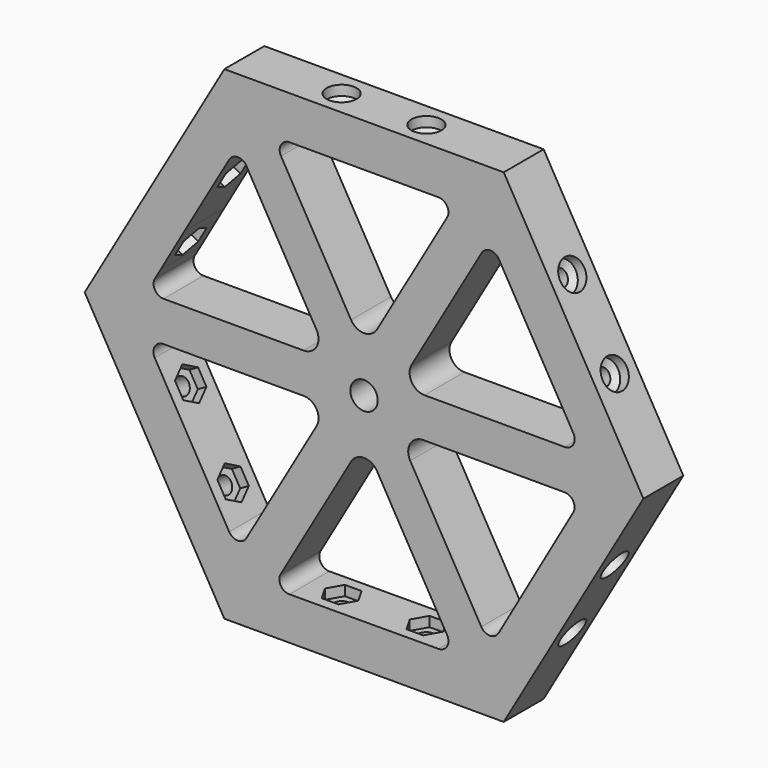
from build123d import *

# Parameters (mm, degrees)
F0_R      = 4
F1_DEPTH  = 3
F2_DEPTH  = 10
F8_D      = 6
F8_DEPTH  = 2
F8_TIP    = 1.8025818571
F9_D      = 3.3
F9_DEPTH  = 13.5
F9_START  = 2.8111618
F9_TIP    = 0.9914200214
F10_D     = 3.3
F10_DEPTH = 13.5
F10_TIP   = 0.9914200214
F11_D     = 6
F11_DEPTH = 2
F11_TIP   = 1.8025818571
F12_D     = 6
F12_DEPTH = 2
F12_TIP   = 1.8025818571
F13_D     = 3.3
F13_DEPTH = 13.5
F13_START = 2.8111618
F13_TIP   = 0.9914200214
F15_D     = 3.3
F15_DEPTH = 13.5
F15_TIP   = 0.9914200214
F16_D     = 6
F16_DEPTH = 2
F16_TIP   = 1.8025818571
F17_D     = 6
F17_DEPTH = 2
F17_TIP   = 1.8025818571
F18_D     = 3.3
F18_DEPTH = 13.5
F18_START = 2.8111618
F18_TIP   = 0.9914200214
F19_D     = 3.3
F19_DEPTH = 13.5
F19_TIP   = 0.9914200214
F20_D     = 6
F20_DEPTH = 2
F20_TIP   = 1.8025818571
F22_DEPTH = 2
F24_DEPTH = 2
F25_R     = 1.65
F26_DEPTH = 2
F28_DEPTH = 2
F29_R     = 1.65
F30_DEPTH = 2
F32_DEPTH = 2
F34_DEPTH = 2
F35_D     = 5.5
F35_DEPTH = 15.81
F35_TIP   = 1.6523667023


# Not quite as in the source:
# - a feature names something its author has since deleted; it is built from what else it names


with BuildPart() as f1:
    # F0 (on Front) → F1 (new body)
    with BuildSketch(Plane.XZ):
        Polygon((28, -48.4974226119), (56, 0), (28, 48.4974226119), (-28, 48.4974226119), (-56, 0), (-28, -48.4974226119), align=None)
        with BuildLine():
            ThreePointArc((-2.5980762114, -12.5), (0, -11), (2.5980762114, -12.5))
            Line((2.5980762114, -12.5), (16.6589147242, -36.8540867013))
            ThreePointArc((16.6589147242, -36.8540867013), (16.6605005999, -38.8513348401), (14.9332161477, -39.8540766136))
            Line((14.9332161477, -39.8540766136), (-14.9735632922, -39.9490644792))
            ThreePointArc((-14.9735632922, -39.9490644792), (-16.7117197395, -38.9526061697), (-16.7137597469, -36.9490810672))
            Line((-16.7137597469, -36.9490810672), (-2.5980762114, -12.5))
        make_face(mode=Mode.SUBTRACT)
        with BuildLine():
            ThreePointArc((-23.5773502692, -32.8371685741), (-25.3094010768, -33.8371685741), (-27.0414518843, -32.8371685741))
            Line((-27.0414518843, -32.8371685741), (-41.9585481157, -7))
            ThreePointArc((-41.9585481157, -7), (-41.9585481157, -5), (-40.2264973081, -4))
            Line((-40.2264973081, -4), (-12.124355653, -4))
            ThreePointArc((-12.124355653, -4), (-9.5262794416, -5.5), (-9.5262794416, -8.5))
            Line((-9.5262794416, -8.5), (-23.5773502692, -32.8371685741))
        make_face(mode=Mode.SUBTRACT)
        with BuildLine():
            ThreePointArc((40.196294044, -4), (41.9262006049, -4.9962952173), (41.9326095328, -6.9925767092))
            Line((41.9326095328, -6.9925767092), (26.9692910507, -33.1679255788))
            ThreePointArc((26.9692910507, -33.1679255788), (25.2372561213, -34.1753442888), (23.5009247544, -33.1753488696))
            Line((23.5009247544, -33.1753488696), (9.2546054422, -8.5))
            ThreePointArc((9.2546054422, -8.5), (9.2546054422, -5.5), (11.8526816536, -4))
            Line((11.8526816536, -4), (40.196294044, -4))
        make_face(mode=Mode.SUBTRACT)
        Circle(F0_R, mode=Mode.SUBTRACT)
        with BuildLine():
            Line((-40.714927966, 9.0731171196), (-35.9903810568, 17.3371685741))
            Line((-35.9903810568, 17.3371685741), (-27.0414518843, 32.8371685741))
            ThreePointArc((-27.0414518843, 32.8371685741), (-25.3094010768, 33.8371685741), (-23.5773502692, 32.8371685741))
            Line((-23.5773502692, 32.8371685741), (-9.5262794416, 8.5))
            ThreePointArc((-9.5262794416, 8.5), (-9.5262794416, 5.5), (-12.124355653, 4))
            Line((-12.124355653, 4), (-40.1904464376, 4))
            ThreePointArc((-40.1904464376, 4), (-41.9244201051, 5.0033379106), (-41.918632256, 7.0066646796))
            Line((-41.918632256, 7.0066646796), (-40.714927966, 9.0731171196))
        make_face(mode=Mode.SUBTRACT)
        with BuildLine():
            Line((40.2264973081, 4), (12.124355653, 4))
            ThreePointArc((12.124355653, 4), (9.5262794416, 5.5), (9.5262794416, 8.5))
            Line((9.5262794416, 8.5), (23.5773502692, 32.8371685741))
            ThreePointArc((23.5773502692, 32.8371685741), (25.3094010768, 33.8371685741), (27.0414518843, 32.8371685741))
            Line((27.0414518843, 32.8371685741), (41.9585481157, 7))
            ThreePointArc((41.9585481157, 7), (41.9585481157, 5), (40.2264973081, 4))
        make_face(mode=Mode.SUBTRACT)
        with BuildLine():
            ThreePointArc((-16.6491470389, 36.8371685741), (-16.6491470389, 38.8371685741), (-14.9170962313, 39.8371685741))
            Line((-14.9170962313, 39.8371685741), (14.9170962313, 39.8371685741))
            ThreePointArc((14.9170962313, 39.8371685741), (16.6491470389, 38.8371685741), (16.6491470389, 36.8371685741))
            Line((16.6491470389, 36.8371685741), (2.5980762114, 12.5))
            ThreePointArc((2.5980762114, 12.5), (0, 11), (-2.5980762114, 12.5))
            Line((-2.5980762114, 12.5), (-16.6491470389, 36.8371685741))
        make_face(mode=Mode.SUBTRACT)
        Circle(F0_R)
    extrude(amount=F1_DEPTH)

    # F0 (on Front) → F2 (join)
    with BuildSketch(Plane.XZ):
        Polygon((28, -48.4974226119), (56, 0), (28, 48.4974226119), (-28, 48.4974226119), (-56, 0), (-28, -48.4974226119), align=None)
        with BuildLine():
            ThreePointArc((-2.5980762114, -12.5), (0, -11), (2.5980762114, -12.5))
            Line((2.5980762114, -12.5), (16.6589147242, -36.8540867013))
            ThreePointArc((16.6589147242, -36.8540867013), (16.6605005999, -38.8513348401), (14.9332161477, -39.8540766136))
            Line((14.9332161477, -39.8540766136), (-14.9735632922, -39.9490644792))
            ThreePointArc((-14.9735632922, -39.9490644792), (-16.7117197395, -38.9526061697), (-16.7137597469, -36.9490810672))
            Line((-16.7137597469, -36.9490810672), (-2.5980762114, -12.5))
        make_face(mode=Mode.SUBTRACT)
        with BuildLine():
            ThreePointArc((-23.5773502692, -32.8371685741), (-25.3094010768, -33.8371685741), (-27.0414518843, -32.8371685741))
            Line((-27.0414518843, -32.8371685741), (-41.9585481157, -7))
            ThreePointArc((-41.9585481157, -7), (-41.9585481157, -5), (-40.2264973081, -4))
            Line((-40.2264973081, -4), (-12.124355653, -4))
            ThreePointArc((-12.124355653, -4), (-9.5262794416, -5.5), (-9.5262794416, -8.5))
            Line((-9.5262794416, -8.5), (-23.5773502692, -32.8371685741))
        make_face(mode=Mode.SUBTRACT)
        with BuildLine():
            ThreePointArc((40.196294044, -4), (41.9262006049, -4.9962952173), (41.9326095328, -6.9925767092))
            Line((41.9326095328, -6.9925767092), (26.9692910507, -33.1679255788))
            ThreePointArc((26.9692910507, -33.1679255788), (25.2372561213, -34.1753442888), (23.5009247544, -33.1753488696))
            Line((23.5009247544, -33.1753488696), (9.2546054422, -8.5))
            ThreePointArc((9.2546054422, -8.5), (9.2546054422, -5.5), (11.8526816536, -4))
            Line((11.8526816536, -4), (40.196294044, -4))
        make_face(mode=Mode.SUBTRACT)
        Circle(F0_R, mode=Mode.SUBTRACT)
        with BuildLine():
            Line((-40.714927966, 9.0731171196), (-35.9903810568, 17.3371685741))
            Line((-35.9903810568, 17.3371685741), (-27.0414518843, 32.8371685741))
            ThreePointArc((-27.0414518843, 32.8371685741), (-25.3094010768, 33.8371685741), (-23.5773502692, 32.8371685741))
            Line((-23.5773502692, 32.8371685741), (-9.5262794416, 8.5))
            ThreePointArc((-9.5262794416, 8.5), (-9.5262794416, 5.5), (-12.124355653, 4))
            Line((-12.124355653, 4), (-40.1904464376, 4))
            ThreePointArc((-40.1904464376, 4), (-41.9244201051, 5.0033379106), (-41.918632256, 7.0066646796))
            Line((-41.918632256, 7.0066646796), (-40.714927966, 9.0731171196))
        make_face(mode=Mode.SUBTRACT)
        with BuildLine():
            Line((40.2264973081, 4), (12.124355653, 4))
            ThreePointArc((12.124355653, 4), (9.5262794416, 5.5), (9.5262794416, 8.5))
            Line((9.5262794416, 8.5), (23.5773502692, 32.8371685741))
            ThreePointArc((23.5773502692, 32.8371685741), (25.3094010768, 33.8371685741), (27.0414518843, 32.8371685741))
            Line((27.0414518843, 32.8371685741), (41.9585481157, 7))
            ThreePointArc((41.9585481157, 7), (41.9585481157, 5), (40.2264973081, 4))
        make_face(mode=Mode.SUBTRACT)
        with BuildLine():
            ThreePointArc((-16.6491470389, 36.8371685741), (-16.6491470389, 38.8371685741), (-14.9170962313, 39.8371685741))
            Line((-14.9170962313, 39.8371685741), (14.9170962313, 39.8371685741))
            ThreePointArc((14.9170962313, 39.8371685741), (16.6491470389, 38.8371685741), (16.6491470389, 36.8371685741))
            Line((16.6491470389, 36.8371685741), (2.5980762114, 12.5))
            ThreePointArc((2.5980762114, 12.5), (0, 11), (-2.5980762114, 12.5))
            Line((-2.5980762114, 12.5), (-16.6491470389, 36.8371685741))
        make_face(mode=Mode.SUBTRACT)
        Circle(F0_R)
    extrude(amount=F2_DEPTH)

    # F8
    with Locations(Plane(origin=(0, 0, -48.4974226119), x_dir=(1, 0, 0), z_dir=(0, 0, -1))):
        with Locations((-8.5, 5), (8.5, 5)):
            Hole(F8_D / 2, depth=F8_DEPTH)
            with Locations((0, 0, -(F8_DEPTH + F8_TIP / 2))):  # 118° drill point
                Cone(0, F8_D / 2, F8_TIP, mode=Mode.SUBTRACT)

    # F9
    # its depths count from where the whole tool has entered the part; down to there all is cleared
    with Locations(Plane(origin=(0, 0, -48.4974226119), x_dir=(1, 0, 0), z_dir=(0, 0, -1)).offset(-F9_START)):
        with Locations((-8.5, 5), (8.5, 5)):
            Hole(F9_D / 2, depth=F9_DEPTH)
            with Locations((0, 0, -(F9_DEPTH + F9_TIP / 2))):  # 118° drill point
                Cone(0, F9_D / 2, F9_TIP, mode=Mode.SUBTRACT)

    # F10
    with Locations(Plane(origin=(42, 0, -24.248711306), x_dir=(0, 1, 0), z_dir=(0.8660254038, 0, -0.5))):
        with Locations((-5, -8.5), (-5, 8.5)):
            Hole(F10_D / 2, depth=F10_DEPTH)
            with Locations((0, 0, -(F10_DEPTH + F10_TIP / 2))):  # 118° drill point
                Cone(0, F10_D / 2, F10_TIP, mode=Mode.SUBTRACT)

    # F11
    with Locations(Plane(origin=(42, 0, -24.248711306), x_dir=(0, 1, 0), z_dir=(0.8660254038, 0, -0.5))):
        with Locations((-5, -8.5), (-5, 8.5)):
            Hole(F11_D / 2, depth=F11_DEPTH)
            with Locations((0, 0, -(F11_DEPTH + F11_TIP / 2))):  # 118° drill point
                Cone(0, F11_D / 2, F11_TIP, mode=Mode.SUBTRACT)

    # F12
    with Locations(Plane(origin=(42, 0, 24.248711306), x_dir=(0, 1, 0), z_dir=(0.8660254038, 0, 0.5))):
        with Locations((-4.9999787869, -8.5), (-4.9999602934, 8.5)):
            Hole(F12_D / 2, depth=F12_DEPTH)
            with Locations((0, 0, -(F12_DEPTH + F12_TIP / 2))):  # 118° drill point
                Cone(0, F12_D / 2, F12_TIP, mode=Mode.SUBTRACT)

    # F13
    # its depths count from where the whole tool has entered the part; down to there all is cleared
    with Locations(Plane(origin=(42, 0, 24.248711306), x_dir=(0, 1, 0), z_dir=(0.8660254038, 0, 0.5)).offset(-F13_START)):
        with Locations((-4.9999787869, -8.5), (-4.9999602934, 8.5)):
            Hole(F13_D / 2, depth=F13_DEPTH)
            with Locations((0, 0, -(F13_DEPTH + F13_TIP / 2))):  # 118° drill point
                Cone(0, F13_D / 2, F13_TIP, mode=Mode.SUBTRACT)

    # F15
    with Locations(Plane.XY.offset(48.4974226119)):
        with Locations((8.5, -5), (-8.5, -5)):
            Hole(F15_D / 2, depth=F15_DEPTH)
            with Locations((0, 0, -(F15_DEPTH + F15_TIP / 2))):  # 118° drill point
                Cone(0, F15_D / 2, F15_TIP, mode=Mode.SUBTRACT)

    # F16
    with Locations(Plane.XY.offset(48.4974226119)):
        with Locations((8.5, -5), (-8.5, -5)):
            Hole(F16_D / 2, depth=F16_DEPTH)
            with Locations((0, 0, -(F16_DEPTH + F16_TIP / 2))):  # 118° drill point
                Cone(0, F16_D / 2, F16_TIP, mode=Mode.SUBTRACT)

    # F17
    with Locations(Plane(origin=(-42, 0, 24.248711306), x_dir=(0, -1, 0), z_dir=(-0.8660254038, 0, 0.5))):
        with Locations((5, 8.5), (5, -8.5)):
            Hole(F17_D / 2, depth=F17_DEPTH)
            with Locations((0, 0, -(F17_DEPTH + F17_TIP / 2))):  # 118° drill point
                Cone(0, F17_D / 2, F17_TIP, mode=Mode.SUBTRACT)

    # F18
    # its depths count from where the whole tool has entered the part; down to there all is cleared
    with Locations(Plane(origin=(-42, 0, 24.248711306), x_dir=(0, -1, 0), z_dir=(-0.8660254038, 0, 0.5)).offset(-F18_START)):
        with Locations((5, 8.5), (5, -8.5)):
            Hole(F18_D / 2, depth=F18_DEPTH)
            with Locations((0, 0, -(F18_DEPTH + F18_TIP / 2))):  # 118° drill point
                Cone(0, F18_D / 2, F18_TIP, mode=Mode.SUBTRACT)

    # F19
    with Locations(Plane(origin=(-42, 0, -24.248711306), x_dir=(0, -1, 0), z_dir=(-0.8660254038, 0, -0.5))):
        with Locations((5, 8.5), (5, -8.5)):
            Hole(F19_D / 2, depth=F19_DEPTH)
            with Locations((0, 0, -(F19_DEPTH + F19_TIP / 2))):  # 118° drill point
                Cone(0, F19_D / 2, F19_TIP, mode=Mode.SUBTRACT)

    # F20
    with Locations(Plane(origin=(-42, 0, -24.248711306), x_dir=(0, -1, 0), z_dir=(-0.8660254038, 0, -0.5))):
        with Locations((5, 8.5), (5, -8.5)):
            Hole(F20_D / 2, depth=F20_DEPTH)
            with Locations((0, 0, -(F20_DEPTH + F20_TIP / 2))):  # 118° drill point
                Cone(0, F20_D / 2, F20_TIP, mode=Mode.SUBTRACT)

    # F21 (on face) → F22 (cut)
    with BuildSketch(Plane(origin=(34.5, 0, 19.918584287), x_dir=(0, -1, 0), z_dir=(-0.8660254038, 0, -0.5))):
        Polygon((4.9999602934, 5.1513684387), (7.8999602934, 6.8256842194), (7.8999602934, 10.1743157806), (4.9999602934, 11.8486315613), (2.0999602934, 10.1743157806), (2.0999602934, 6.8256842194), align=None)
        Polygon((2.0999787869, -10.1743157807), (4.9999787869, -11.8486315613), (7.8999787869, -10.1743157807), (7.8999787869, -6.8256842194), (4.9999787869, -5.1513684387), (2.0999787869, -6.8256842194), align=None)
    extrude(amount=-F22_DEPTH, mode=Mode.SUBTRACT)

    # F23 (on face) → F24 (cut)
    with BuildSketch(Plane(origin=(0, 0, 39.8371685741), x_dir=(1, 0, 0), z_dir=(0, 0, -1))):
        Polygon((10.1743157806, 7.9), (6.8256842194, 7.9), (5.1513684387, 5), (6.8256842194, 2.1), (10.1743157806, 2.1), (11.8486315613, 5), align=None)
        Polygon((-6.8256842194, 7.9), (-10.1743157806, 7.9), (-11.8486315613, 5), (-10.1743157806, 2.1), (-6.8256842194, 2.1), (-5.1513684387, 5), align=None)
    extrude(amount=-F24_DEPTH, mode=Mode.SUBTRACT)

    # F25 (on face) → F26 (cut)
    with BuildSketch(Plane(origin=(-34.5, 0, 19.918584287), x_dir=(0, 1, 0), z_dir=(0.8660254038, 0, -0.5))):
        Polygon((-4.9822457848, 11.8485844952), (-7.8910821319, 10.189667849), (-7.9088363471, 6.8410833538), (-5.0177542152, 5.1514155048), (-2.1089178681, 6.810332151), (-2.0911636529, 10.1589166462), align=None)
        with Locations((-5, 8.5)):
            Circle(F25_R, mode=Mode.SUBTRACT)
    extrude(amount=-F26_DEPTH, mode=Mode.SUBTRACT)

    # F27 (on face) → F28 (cut)
    with BuildSketch(Plane(origin=(-34.5950076436, 0, 19.7779185352), x_dir=(0, 1, 0), z_dir=(0.86814213, 0, -0.4963156679))):
        Polygon((-7.9, -6.6564354882), (-7.9, -10.0050670495), (-5, -11.6793828301), (-2.1, -10.0050670495), (-2.1, -6.6564354882), (-5, -4.9821197075), align=None)
    extrude(amount=-F28_DEPTH, mode=Mode.SUBTRACT)

    # F29 (on face) → F30 (cut)
    with BuildSketch(Plane(origin=(-34.5, 0, -19.918584287), x_dir=(0, 1, 0), z_dir=(0.8660254038, 0, 0.5))):
        Polygon((-7.9, -6.8256842194), (-7.9, -10.1743157806), (-5, -11.8486315613), (-2.1, -10.1743157806), (-2.1, -6.8256842194), (-5, -5.1513684387), align=None)
        with Locations((-5, -8.5)):
            Circle(F29_R, mode=Mode.SUBTRACT)
        Polygon((-7.9, 10.1743157806), (-7.9, 6.8256842194), (-5, 5.1513684387), (-2.1, 6.8256842194), (-2.1, 10.1743157806), (-5, 11.8486315613), align=None)
        with Locations((-5, 8.5)):
            Circle(F29_R, mode=Mode.SUBTRACT)
    extrude(amount=-F30_DEPTH, mode=Mode.SUBTRACT)

    # F31 (on face) → F32 (cut)
    with BuildSketch(Plane(origin=(0.1267311551, 0, -39.9011039577), x_dir=(0.9999949561, 0, 0.0031761155), z_dir=(-0.0031761155, 0, 0.9999949561))):
        Polygon((5.0247066547, -5.0134812621), (6.7106839822, -7.9067171295), (10.0592884063, -7.8932358674), (11.7219155029, -4.9865187379), (10.0359381754, -2.0932828705), (6.6873337513, -2.1067641326), align=None)
        Polygon((-10.301090448, -7.9), (-6.9524588867, -7.9), (-5.2781431061, -5), (-6.9524588867, -2.1), (-10.301090448, -2.1), (-11.9754062287, -5), align=None)
    extrude(amount=-F32_DEPTH, mode=Mode.SUBTRACT)

    # F33 (on face) → F34 (cut)
    with BuildSketch(Plane(origin=(34.617316126, 0, -19.789227214), x_dir=(0, -1, 0), z_dir=(-0.8681577444, 0, 0.4962883546))):
        Polygon((7.9, -10.3450797931), (7.9, -6.9964482318), (5, -5.3221324512), (2.1, -6.9964482318), (2.1, -10.3450797931), (5, -12.0193955738), align=None)
        Polygon((7.9, 6.6550759554), (7.9, 10.0037075167), (5, 11.6780232974), (2.1, 10.0037075167), (2.1, 6.6550759554), (5, 4.9807601748), align=None)
    extrude(amount=-F34_DEPTH, mode=Mode.SUBTRACT)

    # F35
    with Locations(Plane(origin=(0, 0, 0), x_dir=(1, 0, 0), z_dir=(0, 1, 0))):
        with Locations((0, 0)):
            Hole(F35_D / 2, depth=F35_DEPTH)
            with Locations((0, 0, -(F35_DEPTH + F35_TIP / 2))):  # 118° drill point
                Cone(0, F35_D / 2, F35_TIP, mode=Mode.SUBTRACT)


solid = f1.part
